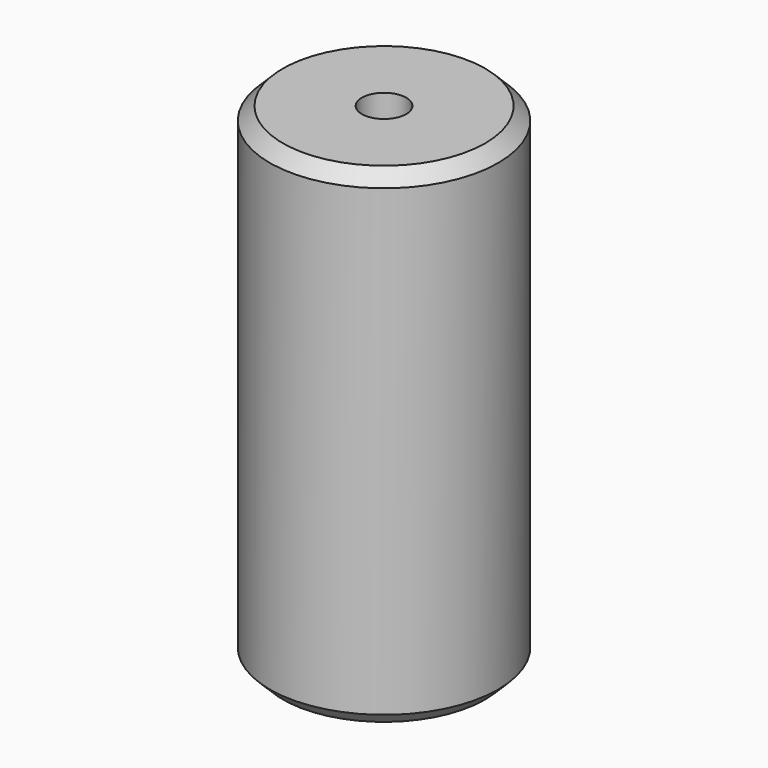
from build123d import *

# Parameters (mm, degrees)
F0_R      = 17.5
F1_DEPTH  = 37.5
F2_R      = 4.25
F3_DEPTH  = 25
F4_SIZE   = 2
F6_R      = 17.5
F7_DEPTH  = 37.5
F8_R      = 4.25
F9_DEPTH  = 30
F10_SIZE  = 2
F11_R     = 5.5
F11_R_2   = 3.4
F12_DEPTH = 30


with BuildPart() as f1:
    # F0 (on Top) → F1 (new body, symmetric)
    with BuildSketch(Plane.XY):
        Circle(F0_R)
    extrude(amount=F1_DEPTH, both=True)

    # F2 (on face) → F3 (cut)
    with BuildSketch(Plane.XY.offset(37.5)):
        Circle(F2_R)
    extrude(amount=-F3_DEPTH, mode=Mode.SUBTRACT)

    # F4
    f4_edges = [f1.edges().sort_by_distance(p)[0] for p in [
        (-17.5, 0, 37.5),
        (-17.5, 0, -37.5),
    ]]
    chamfer(f4_edges, length=F4_SIZE)


with BuildPart() as f7:
    # F6 (on Top) → F7 (new body, symmetric)
    with BuildSketch(Plane.XY):
        Circle(F6_R)
    extrude(amount=F7_DEPTH, both=True)

    # F8 (on face) → F9 (cut)
    with BuildSketch(Plane.XY.offset(37.5)):
        Circle(F8_R)
    extrude(amount=-F9_DEPTH, mode=Mode.SUBTRACT)

    # F10
    f10_edges = [f7.edges().sort_by_distance(p)[0] for p in [
        (-17.5, 0, 37.5),
        (-17.5, 0, -37.5),
    ]]
    chamfer(f10_edges, length=F10_SIZE)

    # F11 (on face) → F12 (join)
    with BuildSketch(Plane.XY.offset(37.5)):
        Circle(F11_R)
        Circle(F11_R_2, mode=Mode.SUBTRACT)
    extrude(amount=-F12_DEPTH)


solid = f7.part
